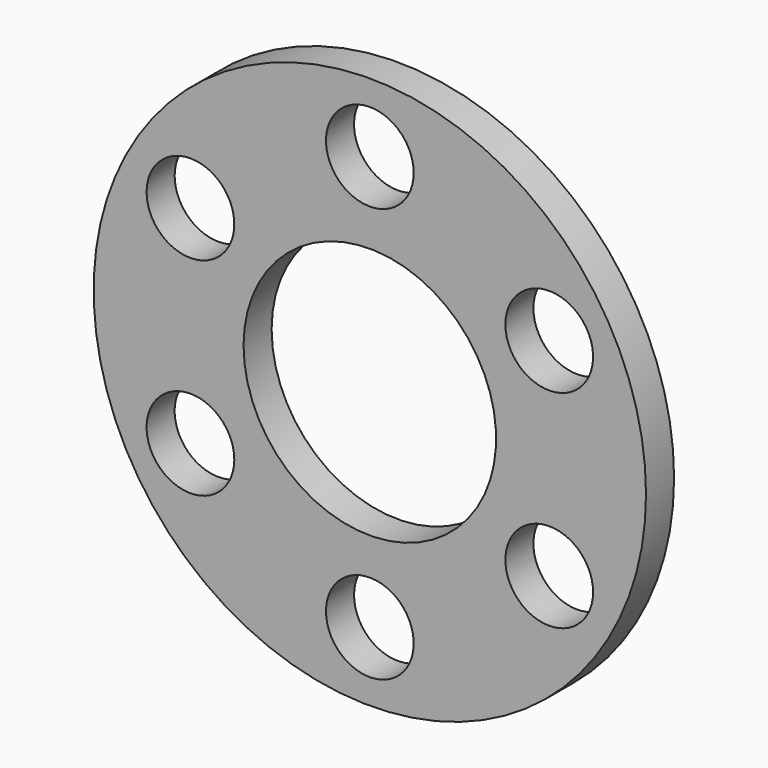
from build123d import *

# Parameters (mm, degrees)
F0_R            = 20
F1_DEPTH        = 2.54
F2_R            = 9.144
F3_DEPTH        = 8.5
F4_R            = 3.175
F5_DEPTH        = 2.541
F5_COPIES_COUNT = 6


# Not quite as in the source:
# - a pattern or mirror of a feature is missing from the dataset's text; its kind, count and spacing are read off the source's solid


with BuildPart() as f1:
    # F0 (on Front) → F1 (new body)
    with BuildSketch(Plane.XZ):
        Circle(F0_R)
    extrude(amount=F1_DEPTH)

    # F2 (on face) → F3 (cut)
    with BuildSketch(Plane(origin=(0, 0, 0), x_dir=(-1, 0, 0), z_dir=(0, 1, 0))):
        Circle(F2_R)
    extrude(amount=-F3_DEPTH, mode=Mode.SUBTRACT)

    # F4 (on face) → F5 (cut, through all)
    with BuildSketch(Plane.XZ.offset(2.54)):
        with Locations((0, 15)):
            Circle(F4_R)
    f5 = extrude(amount=-F5_DEPTH, mode=Mode.SUBTRACT)

    # F5_copies: F5 ×6 about axis
    f5_copies_axis = Axis((0, 0, 0), (0, 1, 0))
    for i in range(1, F5_COPIES_COUNT):
        add(f5.rotate(f5_copies_axis, i * 360 / F5_COPIES_COUNT), mode=Mode.SUBTRACT)


solid = f1.part
